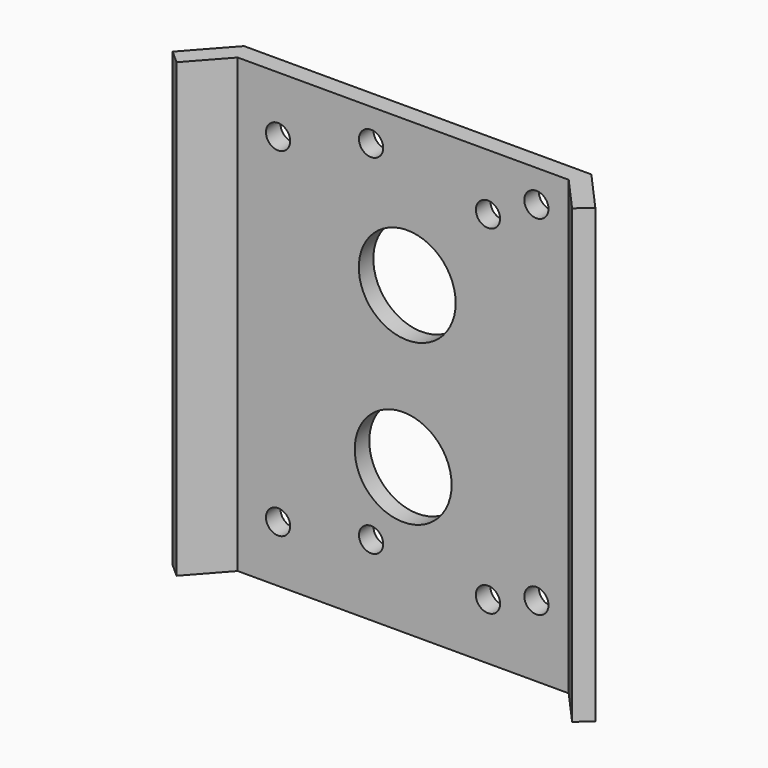
from build123d import *

# Parameters (mm, degrees)
F1_DEPTH = 88.9
F3_D     = 19.05
F5_D     = 4.7625


# Not quite as in the source:
# - a feature names something its author has since deleted; it is built from what else it names


with BuildPart() as f1:
    # F0 (on Top) → F1 (new body)
    with BuildSketch(Plane.XY):
        Polygon((10.538799933, 10.6713908286), (-57.7562613184, 10.6713908286), (-65.16550908, 2.3876), (-62.4960911285, 0), (-56.1460911285, 7.0995158286), (8.9414088715, 7.0995158286), (15.2914088715, 0), (17.9537273073, 2.38125), align=None)
    extrude(amount=F1_DEPTH)

    # F3 (through all)
    with Locations(Plane(origin=(0, 10.6713908286, 0), x_dir=(-1, 0, 0), z_dir=(0, 1, 0))):
        with Locations((22.8085911285, 60.325), (23.6087306927, 28.575)):
            Hole(F3_D / 2)

    # F5 (through all)
    with Locations(Plane(origin=(0, 10.6713908286, 0), x_dir=(-1, 0, 0), z_dir=(0, 1, 0))):
        with Locations((-2.5914088715, 82.55), (29.9205911285, 82.55), (29.9205911285, 13.97), (-2.5914088715, 13.97), (48.2085911285, 11.0998), (48.2085911285, 77.7748), (6.9335911285, 77.7748), (6.9335911285, 11.0998)):
            Hole(F5_D / 2)


solid = f1.part
